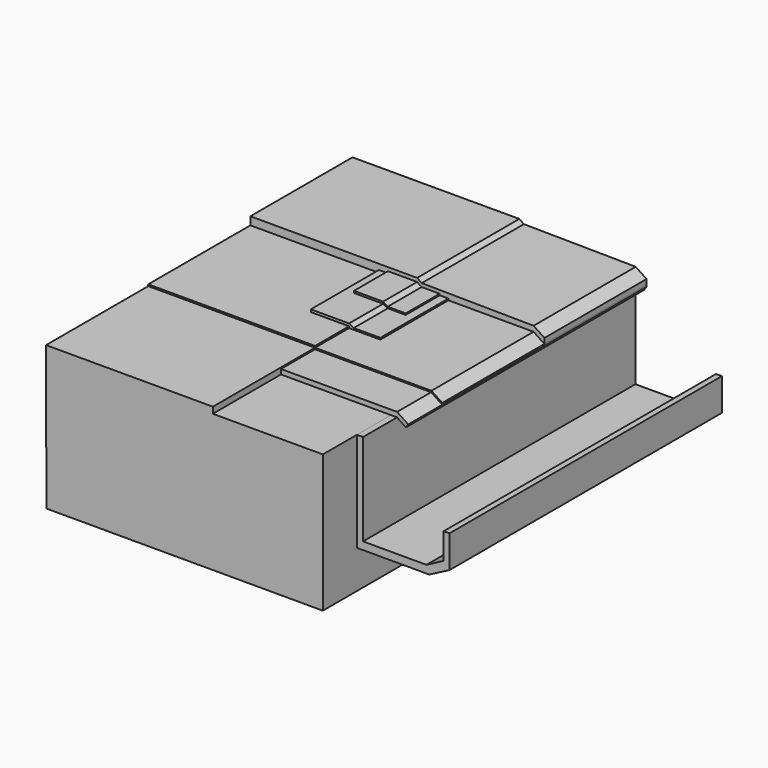
from build123d import *

# Parameters (mm, degrees)
F1_DEPTH = 90
F2_DEPTH = 80
F3_DEPTH = 70
F4_DEPTH = 60
F5_DEPTH = 60
F6_DEPTH = 50
F7_DEPTH = 40
F8_DEPTH = 30


# Not quite as in the source:
# - a feature names something its author has since deleted; it is built from what else it names


with BuildPart() as f1:
    # F0 (on Front) → F1 (new body)
    with BuildSketch(Plane.XZ):
        Polygon((-35.844899714, 19.0136060119), (-75.0298798084, 19.0136060119), (-74.9661251903, -14.775316231), (-9.9985962734, -14.775316231), (-9.9985962734, -5.8398880064), (-9.9985962734, 16.2808988243), (-9.9985962734, 17.5495628755), (-35.844899714, 17.5495628755), (-35.844899714, 18.6878981805), align=None)
    extrude(amount=F1_DEPTH)


with BuildPart() as f2:
    # F0 (on Front) → F2 (new body)
    with BuildSketch(Plane.XZ):
        Polygon((-9.9985962734, 16.2808988243), (-9.9985962734, -5.8398880064), (6.9901682436, -5.8398880064), (11.7682581767, -3.3623597119), (11.7682581767, 4.2471913621), (10.3489141911, 4.1997791268), (10.3489141911, -1.9189424347), (6.350541953, -4.0392908268), (-8.5561517044, -4.0392908268), (-8.5561517044, 17.5495628755), (-9.9985962734, 17.5495628755), align=None)
    extrude(amount=F2_DEPTH)


with BuildPart() as f3:
    # F0 (on Front) → F3 (new body)
    with BuildSketch(Plane.XZ):
        Polygon((-8.5561517044, 18.6878981805), (-35.844899714, 18.6878981805), (-35.844899714, 17.5495628755), (-9.9985962734, 17.5495628755), (-8.5561517044, 17.5495628755), (-6.4736446366, 16.1520168185), (-5.9469314412, 16.9368810786), align=None)
    extrude(amount=F3_DEPTH)


with BuildPart() as f4:
    # F0 (on Front) → F4 (new body)
    with BuildSketch(Plane.XZ):
        Polygon((-75.0298798084, 19.3932503462), (-75.0298798084, 19.0136060119), (-35.844899714, 19.0136060119), (-35.8411632478, 19.3932503462), (-44.8312833905, 19.3932503462), align=None)
    extrude(amount=F4_DEPTH)


with BuildPart() as f5:
    # F0 (on Front) → F5 (new body)
    with BuildSketch(Plane.XZ):
        Polygon((-28.500309214, 19.0136060119), (-35.844899714, 19.0136060119), (-35.844899714, 18.6878981805), (-8.5561517044, 18.6878981805), (-5.9469314412, 16.9368810786), (-5.9469314412, 17.3235815018), (-8.4827402607, 19.0136060119), align=None)
    extrude(amount=F5_DEPTH)


with BuildPart() as f6:
    # F0 (on Front) → F6 (new body)
    with BuildSketch(Plane.XZ):
        Polygon((-35.8411632478, 19.3932503462), (-35.844899714, 19.0136060119), (-28.500309214, 19.0136060119), (-28.500309214, 19.3932503462), (-30.5376388133, 19.3932503462), (-34.7416512668, 19.3932503462), (-35.844899714, 19.9753437191), (-42.6969379187, 19.9753437191), (-44.8312833905, 19.9753437191), (-44.8312833905, 19.3932503462), align=None)
    extrude(amount=F6_DEPTH)


with BuildPart() as f7:
    # F0 (on Front) → F7 (new body)
    with BuildSketch(Plane.XZ):
        Polygon((-34.7416512668, 19.3932503462), (-30.5376388133, 19.3932503462), (-30.5376388133, 19.7169722799), (-34.7852603294, 19.7169722799), (-35.844899714, 20.428083837), (-42.6969379187, 20.428083837), (-42.6969379187, 19.9753437191), (-35.844899714, 19.9753437191), align=None)
    extrude(amount=F7_DEPTH)


with BuildPart() as f8:
    # F0 (on Front) → F8 (new body)
    with BuildSketch(Plane.XZ):
        Polygon((-75.0298798084, 21.2688874453), (-75.0298798084, 19.3932503462), (-44.8312833905, 19.3932503462), (-44.8312833905, 19.9753437191), (-42.6969379187, 19.9753437191), (-42.6969379187, 20.428083837), (-35.844899714, 20.428083837), (-34.7852603294, 19.7169722799), (-30.5376388133, 19.7169722799), (-30.5376388133, 19.3932503462), (-28.500309214, 19.3932503462), (-28.500309214, 19.0136060119), (-8.4827402607, 19.0136060119), (-5.9469314412, 17.3235815018), (-5.9469314412, 18.5646397935), (-8.4827402607, 20.2663913369), (-34.7626654522, 20.5426127312), (-35.844899714, 21.2688874453), align=None)
    extrude(amount=F8_DEPTH)


solid = Compound([f1.part, f2.part, f3.part, f4.part, f5.part, f6.part, f7.part, f8.part])
